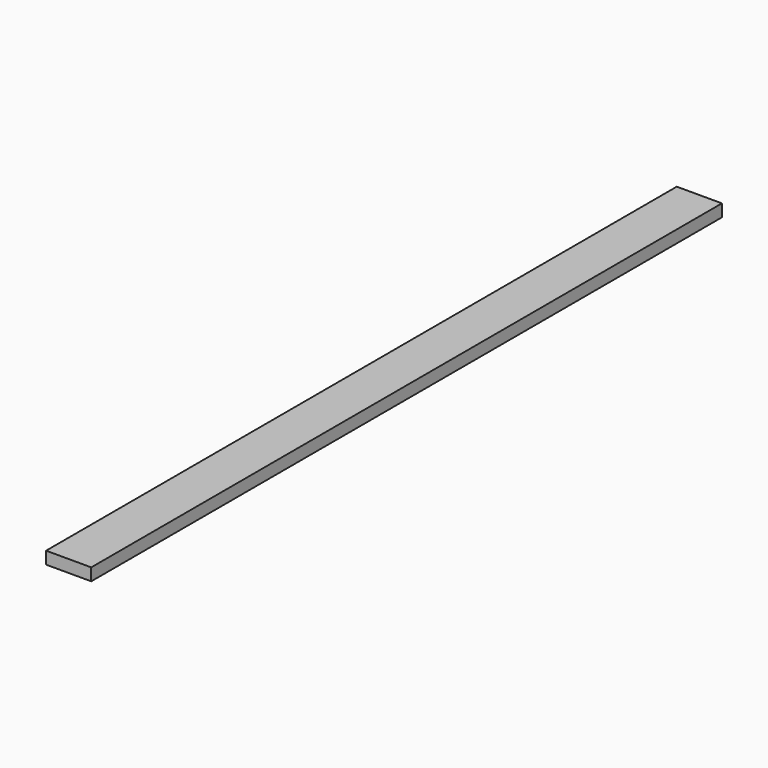
from build123d import *

# Parameters (mm, degrees)
F0_W     = 139.7
F0_H     = 38.1
F2_DEPTH = 1219.2


# Not quite as in the source:
# - a variable given as a bare number and used for a length is read in inches; the dataset says mm whatever the document's units were


with BuildPart() as f2:
    # F0 (on Front) → F2 (new body, symmetric)
    with BuildSketch(Plane.XZ):
        with Locations((-292.1, 742.95)):
            Rectangle(F0_W, F0_H)
    extrude(amount=F2_DEPTH, both=True)


solid = f2.part
